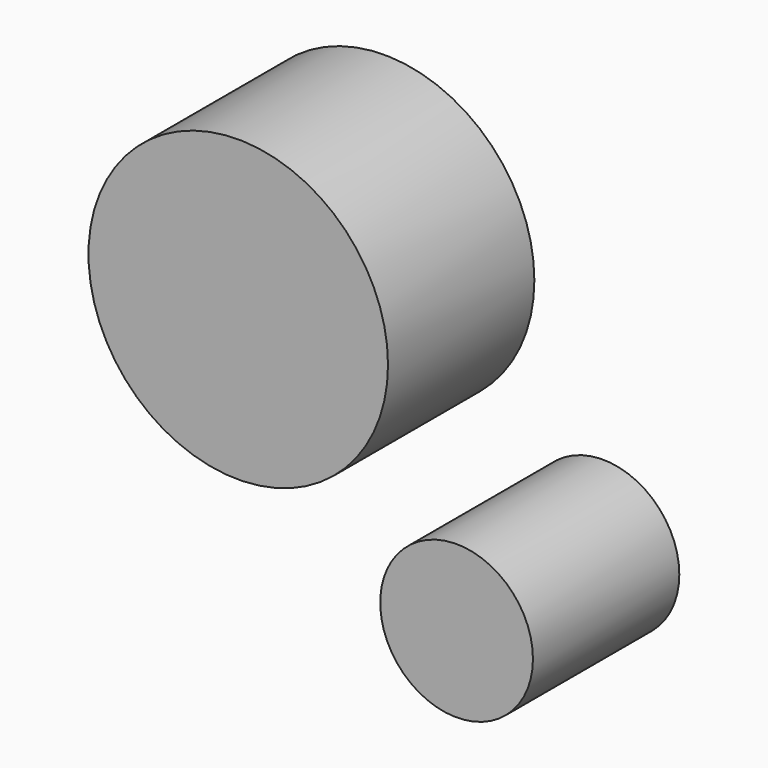
from build123d import *

# Parameters (mm, degrees)
F2_R     = 26.9026463435
F4_DEPTH = 64.4670631737
F1_R     = 18.6019651269
F0_R     = 52.7727745314


with BuildPart() as f4:
    # F2 (on Front) → F4 (new body)
    with BuildSketch(Plane.XZ):
        with Locations((76.9407525659, -74.6546387672)):
            Circle(F2_R)
    extrude(amount=F4_DEPTH)


with BuildPart() as f4b:
    # F1 (on face) → F4, piece 2 (new body)
    with BuildSketch(Plane.XZ):
        Circle(F1_R)
    extrude(amount=F4_DEPTH)


with BuildPart() as f4c:
    # F0 (on Front) → F4, piece 3 (new body)
    with BuildSketch(Plane.XZ):
        Circle(F0_R)
    extrude(amount=F4_DEPTH)


solid = Compound([f4.part, f4b.part, f4c.part])
